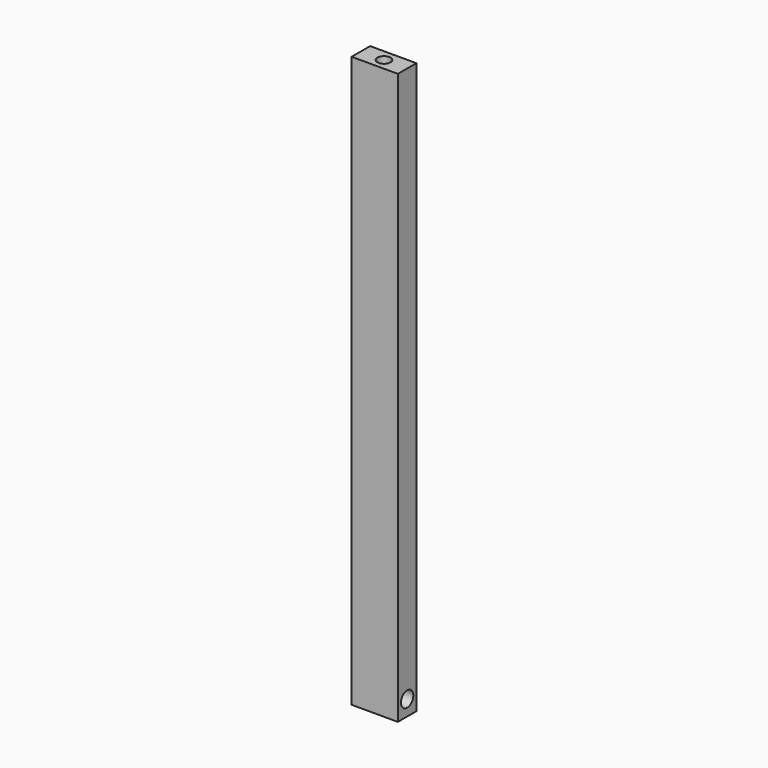
from build123d import *

# Parameters (mm, degrees)
F0_W     = 38.1
F0_H     = 19.05
F1_DEPTH = 234.95
F3_D     = 12.7
F5_D     = 10.71626
F5_DEPTH = 38.1
F5_TIP   = 3.2194893086


# Not quite as in the source:
# - a length typed as a fraction of an inch, garbled in the dataset ("3 / 203.2 mm" for 3/8 in), is restored


with BuildPart() as f1:
    # F0 (on Top) → F1 (new body, symmetric)
    with BuildSketch(Plane.XY):
        Rectangle(F0_W, F0_H)
    extrude(amount=F1_DEPTH, both=True)

    # F3 (through all)
    with Locations(Plane.YZ.offset(19.05)):
        with Locations((0, -222.25)):
            Hole(F3_D / 2)

    # F5
    with Locations(Plane.XY.offset(234.95)):
        with Locations((0, 0)):
            Hole(F5_D / 2, depth=F5_DEPTH)
            with Locations((0, 0, -(F5_DEPTH + F5_TIP / 2))):  # 118° drill point
                Cone(0, F5_D / 2, F5_TIP, mode=Mode.SUBTRACT)


solid = f1.part
